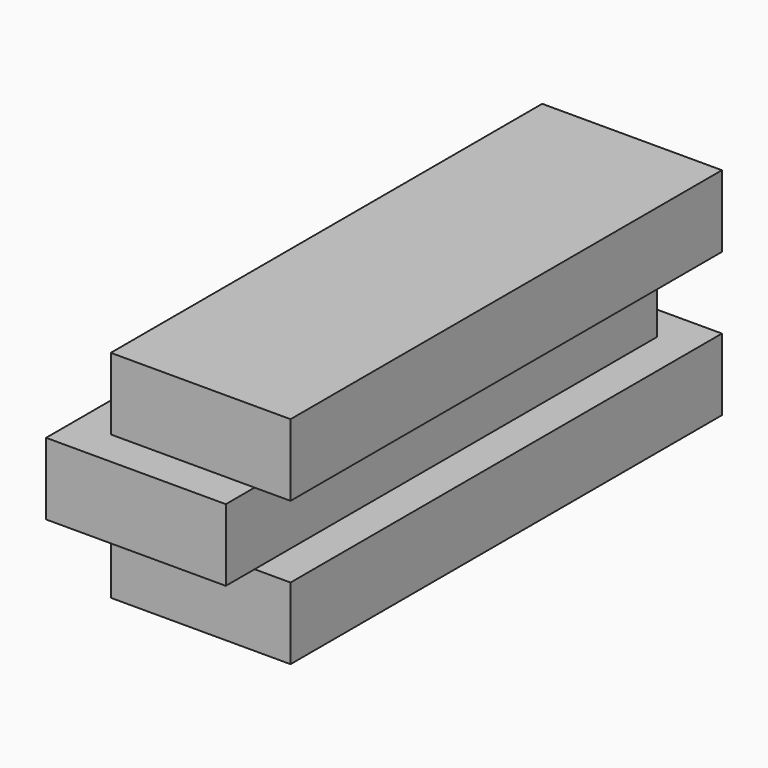
from build123d import *

# Parameters (mm, degrees)
F2_W     = 7.9375
F2_H     = 23.8125
F3_DEPTH = 3.175
F4_W     = 7.9375
F4_H     = 23.8125
F5_DEPTH = 3.175
F6_W     = 7.9375
F6_H     = 23.8125
F7_DEPTH = 3.175


# Not quite as in the source:
# - a variable given as a bare number and used for a length is read in inches; the dataset says mm whatever the document's units were


with BuildPart() as f3:
    # F2 (on Top) → F3 (new body)
    with BuildSketch(Plane.XY):
        with Locations((3.96875, 11.90625)):
            Rectangle(F2_W, F2_H)
    extrude(amount=F3_DEPTH)

    # F4 (on face) → F5 (join)
    with BuildSketch(Plane.XY.offset(3.175)):
        with Locations((2.38125, 10.31875)):
            Rectangle(F4_W, F4_H)
    extrude(amount=F5_DEPTH)

    # F6 (on face) → F7 (join)
    with BuildSketch(Plane.XY.offset(6.35)):
        with Locations((3.96875, 11.90625)):
            Rectangle(F6_W, F6_H)
    extrude(amount=F7_DEPTH)


solid = f3.part
